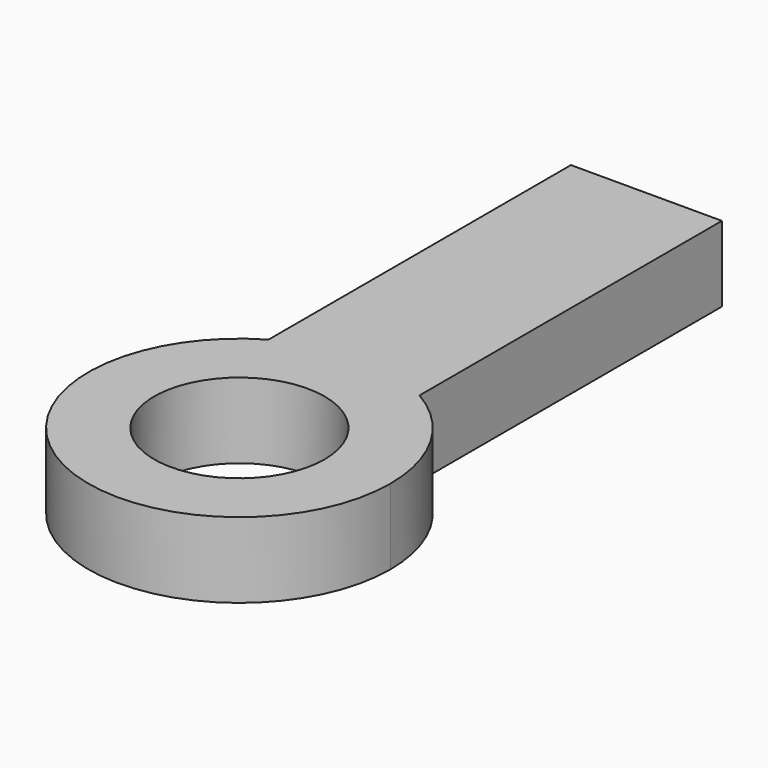
from build123d import *

# Parameters (mm, degrees)
F0_R     = 14.3372968019
F1_DEPTH = 12.7


# Not quite as in the source:
# - a feature names something its author has since deleted; it is built from what else it names


with BuildPart() as f1:
    # F0 (on Top) → F1 (new body)
    with BuildSketch(Plane.XY):
        with BuildLine():
            ThreePointArc((-12.7, 21.9970452561), (0, 25.4), (12.7, 21.9970452561))
            Line((12.7, 21.9970452561), (12.7, 85.5907872319))
            Line((12.7, 85.5907872319), (0, 85.5907872319))
            Line((0, 85.5907872319), (-12.7, 85.5907872319))
            Line((-12.7, 85.5907872319), (-12.7, 21.9970452561))
        make_face()
        with BuildLine():
            ThreePointArc((-12.7, 21.9970452561), (-12.7, -21.9970452561), (25.4, 0))
            ThreePointArc((25.4, 0), (21.9970452561, 12.7), (12.7, 21.9970452561))
            ThreePointArc((12.7, 21.9970452561), (0, 25.4), (-12.7, 21.9970452561))
        make_face()
        Circle(F0_R, mode=Mode.SUBTRACT)
    extrude(amount=F1_DEPTH)


solid = f1.part
